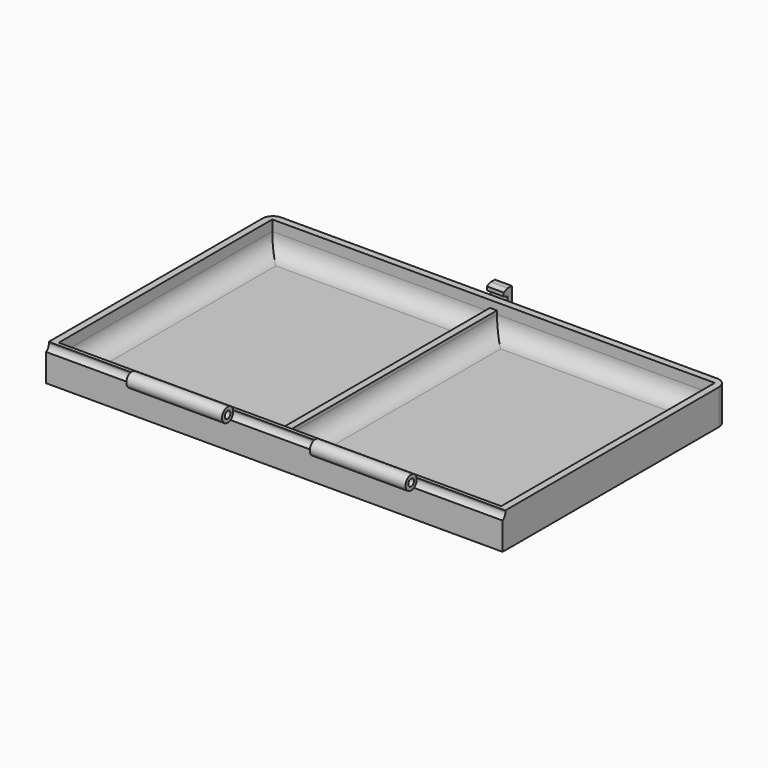
from build123d import *

# Parameters (mm, degrees)
F0_W     = 64
F0_H     = 80
F0_W_2   = 1
F1_DEPTH = 10
F2_T     = -2
F3_DEPTH = 8
F5_DEPTH = 130.001
F6_START = -25.25
F4_R     = 1
F6_DEPTH = 27.25
F8_W     = 1.5
F8_H     = 2
F9_DEPTH = 2.4
F10_R    = 5
F11_R    = 3


# Not quite as in the source:
# - a pattern or mirror of a feature is missing from the dataset's text; its kind, count and spacing are read off the source's solid


with BuildPart() as f1:
    # F0 (on Top) → F1 (new body)
    with BuildSketch(Plane.XY):
        with Locations((-32, 40)):
            Rectangle(F0_W, F0_H)
        with Locations((-64.5, 40)):
            Rectangle(F0_W_2, F0_H)
        with Locations((-65.5, 40)):
            Rectangle(F0_W_2, F0_H)
        with Locations((-98, 40)):
            Rectangle(F0_W, F0_H)
    extrude(amount=F1_DEPTH)

    # F2
    f2_openings = [f1.faces().sort_by_distance(p)[0] for p in [
        (-65, 40, 10),
    ]]
    offset(amount=F2_T, openings=f2_openings)

    # F0 (on Top) → F3 (join)
    with BuildSketch(Plane.XY):
        with Locations((-65.5, 40)):
            Rectangle(F0_W_2, F0_H)
        with Locations((-64.5, 40)):
            Rectangle(F0_W_2, F0_H)
    extrude(amount=F3_DEPTH)

    # F4 (on face) → F5 (cut, through all)
    with BuildSketch(Plane.YZ):
        with BuildLine():
            ThreePointArc((0, 7.8458905733), (0.7245313434, 8.5770948967), (0.9894327009, 9.5717972144))
            ThreePointArc((0.9894327009, 9.5717972144), (0.9778046189, 9.7871506811), (0.9430555853, 10))
            Line((0.9430555853, 10), (0.840551923, 10))
            ThreePointArc((0.840551923, 10), (0.8771729534, 9.7872890681), (0.8894327009, 9.5717972144))
            ThreePointArc((0.8894327009, 9.5717972144), (0.6522733229, 8.6525795765), (0, 7.9628367631))
            Line((0, 7.9628367631), (0, 7.8458905733))
        make_face()
        with BuildLine():
            ThreePointArc((0.8894327009, 9.5717972144), (0.8771729534, 9.7872890681), (0.840551923, 10))
            Line((0.840551923, 10), (0, 10))
            Line((0, 10), (0, 7.9628367631))
            ThreePointArc((0, 7.9628367631), (0.6522733229, 8.6525795765), (0.8894327009, 9.5717972144))
        make_face()
    extrude(amount=-F5_DEPTH, mode=Mode.SUBTRACT)

    # F4 (on face) → F6 (join)
    with BuildSketch(Plane.YZ.offset(F6_START)):
        with BuildLine():
            ThreePointArc((0, 7.8458905733), (0.7245313434, 8.5770948967), (0.9894327009, 9.5717972144))
            ThreePointArc((0.9894327009, 9.5717972144), (0.9778046189, 9.7871506811), (0.9430555853, 10))
            Line((0.9430555853, 10), (0.840551923, 10))
            ThreePointArc((0.840551923, 10), (0.8771729534, 9.7872890681), (0.8894327009, 9.5717972144))
            ThreePointArc((0.8894327009, 9.5717972144), (0.6522733229, 8.6525795765), (0, 7.9628367631))
            Line((0, 7.9628367631), (0, 7.8458905733))
        make_face()
        with BuildLine():
            Line((0.840551923, 10), (0.9430555853, 10))
            ThreePointArc((0.9430555853, 10), (-2.8426843031, 10.3738865383), (0, 7.8458905733))
            Line((0, 7.8458905733), (0, 7.9628367631))
            ThreePointArc((0, 7.9628367631), (-2.7669331351, 10.2964895976), (0.840551923, 10))
        make_face()
        with BuildLine():
            ThreePointArc((0.8894327009, 9.5717972144), (0.8771729534, 9.7872890681), (0.840551923, 10))
            Line((0.840551923, 10), (0, 10))
            Line((0, 10), (0, 7.9628367631))
            ThreePointArc((0, 7.9628367631), (0.6522733229, 8.6525795765), (0.8894327009, 9.5717972144))
        make_face()
        with BuildLine():
            Line((0, 10), (0.840551923, 10))
            ThreePointArc((0.840551923, 10), (-2.7669331351, 10.2964895976), (0, 7.9628367631))
            Line((0, 7.9628367631), (0, 10))
        make_face()
        with Locations((-1.0105672991, 9.5717972144)):
            Circle(F4_R, mode=Mode.SUBTRACT)
    f6 = extrude(amount=-F6_DEPTH)

    # F6_copies: F6 across plane
    add(f6.mirror(Plane(origin=(-65, 0, 0), x_dir=(0, 0, -1), z_dir=(-1, 0, 0))))

    # F8 (on mid) → F9 (join, symmetric)
    with BuildSketch(Plane(origin=(-65, 0, 0), x_dir=(0, -1, 0), z_dir=(-1, 0, 0))):
        Polygon((-80, 13.2), (-80, 11.2), (-78.6, 11.7), (-78.6, 12.7), align=None)
        Polygon((-81.5, 10), (-80, 10), (-80, 11.2), (-80, 13.2), (-81.5, 13.2), align=None)
        with Locations((-80.75, 9)):
            Rectangle(F8_W, F8_H)
    extrude(amount=F9_DEPTH, both=True)

    # F10
    f10_edges = [f1.edges().sort_by_distance(p)[0] for p in [
        (-33, 2, 2),
        (-64, 40, 2),
        (-33, 78, 2),
        (-2, 40, 2),
        (-97, 2, 2),
        (-128, 40, 2),
        (-97, 78, 2),
        (-66, 40, 2),
    ]]
    fillet(f10_edges, radius=F10_R)

    # F11
    f11_edges = [f1.edges().sort_by_distance(p)[0] for p in [
        (-130, 80, 5),
        (0, 80, 5),
    ]]
    fillet(f11_edges, radius=F11_R)


solid = f1.part
